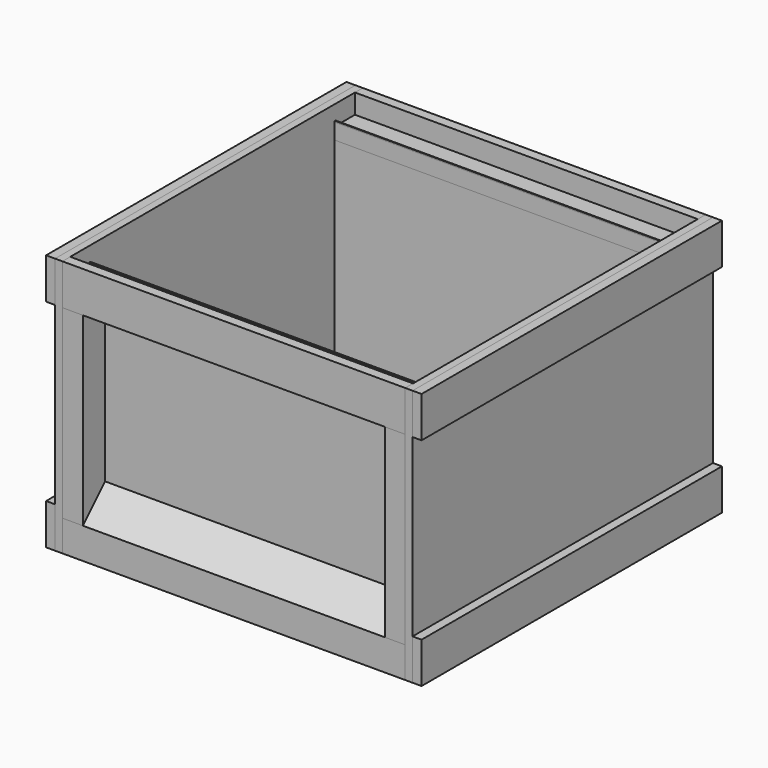
from build123d import *

# Parameters (mm, degrees)
F0_W      = 9
F0_H      = 291
F1_DEPTH  = 210
F2_W      = 34
F2_H      = 38
F3_DEPTH  = 210
F5_DEPTH  = 420
F9_DEPTH  = 9
F10_W     = 11
F10_H     = 50
F11_DEPTH = 460
F12_W     = 34
F12_H     = 227
F13_DEPTH = 25
F16_DEPTH = 370


# Not quite as in the source:
# - ends of sketch curves that miss each other by under 0.0002 mm in the source are joined


with BuildPart() as f1:
    # F0 (on Right) → F1 (new body, symmetric)
    with BuildSketch(Plane.YZ):
        with Locations((39.679, 143.4123)):
            Rectangle(F0_W, F0_H)
    extrude(amount=F1_DEPTH, both=True)


with BuildPart() as f1b:
    # F0 (on Right) → F1, piece 2 (new body, symmetric)
    with BuildSketch(Plane.YZ):
        Polygon((427.179, 288.9123), (418.179, 288.9123), (418.179, -2.0877000002), (427.1789405548, -2.0877634065), align=None)
    extrude(amount=F1_DEPTH, both=True)


with BuildPart() as f3:
    # F2 (on Right) → F3 (new body, symmetric)
    with BuildSketch(Plane.YZ):
        with Locations((18.179, 16.9123)):
            Rectangle(F2_W, F2_H)
    extrude(amount=F3_DEPTH, both=True)


with BuildPart() as f3b:
    # F2 (on Right) → F3, piece 2 (new body, symmetric)
    with BuildSketch(Plane.YZ):
        Polygon((13.179, 312.9123), (1.179, 312.9123), (1.179, 262.9123), (35.179, 262.9123), (35.179, 288.9123), (13.179, 288.9123), align=None)
    extrude(amount=F3_DEPTH, both=True)


with BuildPart() as f3c:
    # F2 (on Right) → F3, piece 3 (new body, symmetric)
    with BuildSketch(Plane.YZ):
        Polygon((461.179, 262.9123), (461.179, 312.9123), (449.179, 312.9123), (449.179, 288.9123), (427.179, 288.9123), (427.179, 262.9123), align=None)
    extrude(amount=F3_DEPTH, both=True)


with BuildPart() as f3d:
    # F2 (on Right) → F3, piece 4 (new body, symmetric)
    with BuildSketch(Plane.YZ):
        with Locations((444.179, 16.9123)):
            Rectangle(F2_W, F2_H)
    extrude(amount=F3_DEPTH, both=True)


with BuildPart() as f5:
    # F4 (on face) → F5 (new body, through all)
    with BuildSketch(Plane.YZ.offset(210)):
        with BuildLine():
            ThreePointArc((43.116056405, 294.2939847231), (43.7817730788, 294.4769973335), (44.179, 293.9123))
            Line((44.179, 293.9123), (44.179, 274.5123))
            Line((44.179, 274.5123), (44.729, 274.5123))
            Line((44.729, 274.5123), (44.729, 293.9123))
            ThreePointArc((44.729, 293.9123), (44.5195970607, 294.5739473149), (43.9676484011, 294.9946365559))
            Line((43.9676484011, 294.9946365559), (43.1903515989, 294.9946365559))
            ThreePointArc((43.1903515989, 294.9946365559), (42.9173526851, 294.8528970607), (42.6916914429, 294.6438623859))
            Line((42.6916914429, 294.6438623859), (38.2546350379, 289.2621776628))
            Line((38.2546350379, 289.2621776628), (38.679, 288.9123))
            Line((38.679, 288.9123), (43.116056405, 294.2939847231))
        make_face()
    extrude(amount=-F5_DEPTH)


with BuildPart() as f7_1:
    # F7: instance of F5
    add(f5.part.mirror(Plane(origin=(0, 231.179, 143.4122999999), x_dir=(-1, 0, 0), z_dir=(0, 1, 0))))


with BuildPart() as f9:
    # F8 (on face) → F9 (new body)
    with BuildSketch(Plane.YZ.offset(210)):
        Polygon((1.179, 312.9123), (1.179, -2.0877), (461.179, -2.0877), (461.179, 312.9123), (13.179, 312.9123), align=None)
    extrude(amount=F9_DEPTH)


with BuildPart() as f11:
    # F10 (on face) → F11 (new body, through all)
    with BuildSketch(Plane.XZ.offset(-1.179)):
        with Locations((224.5, 287.9123)):
            Rectangle(F10_W, F10_H)
    extrude(amount=-F11_DEPTH)


with BuildPart() as f11b:
    # F10 (on face) → F11, piece 2 (new body, through all)
    with BuildSketch(Plane.XZ.offset(-1.179)):
        with Locations((224.5, 22.9123)):
            Rectangle(F10_W, F10_H)
    extrude(amount=-F11_DEPTH)


with BuildPart() as f13:
    # F12 (on face) → F13 (new body)
    with BuildSketch(Plane(origin=(210, 0, 0), x_dir=(0, -1, 0), z_dir=(-1, 0, 0))):
        with Locations((-18.179, 149.4123)):
            Rectangle(F12_W, F12_H)
    extrude(amount=F13_DEPTH)


with BuildPart() as f13b:
    # F12 (on face) → F13, piece 2 (new body)
    with BuildSketch(Plane(origin=(210, 0, 0), x_dir=(0, -1, 0), z_dir=(-1, 0, 0))):
        with Locations((-444.179, 149.4123)):
            Rectangle(F12_W, F12_H)
    extrude(amount=F13_DEPTH)


with BuildPart() as f14_1:
    # F14: instance of F9
    add(f9.part.mirror(Plane.YZ))


with BuildPart() as f14_2:
    # F14: instance of F11b
    add(f11b.part.mirror(Plane.YZ))


with BuildPart() as f14_3:
    # F14: instance of F11
    add(f11.part.mirror(Plane.YZ))


with BuildPart() as f14_4:
    # F14: instance of F13
    add(f13.part.mirror(Plane.YZ))


with BuildPart() as f14_5:
    # F14: instance of F13b
    add(f13b.part.mirror(Plane.YZ))


with BuildPart() as f16:
    # F15 (on face) → F16 (new body, through all)
    with BuildSketch(Plane(origin=(185, 0, 0), x_dir=(0, -1, 0), z_dir=(-1, 0, 0))):
        Polygon((-35.179, 69.9123), (-35.179, 35.9123), (-1.179, 35.9123), align=None)
    extrude(amount=F16_DEPTH)


with BuildPart() as f16b:
    # F15 (on face) → F16, piece 2 (new body, through all)
    with BuildSketch(Plane(origin=(185, 0, 0), x_dir=(0, -1, 0), z_dir=(-1, 0, 0))):
        Polygon((-427.179, 35.9123), (-427.179, 69.9123), (-461.179, 35.9123), align=None)
    extrude(amount=F16_DEPTH)


solid = Compound([f1.part, f1b.part, f3.part, f3b.part, f3c.part, f3d.part, f5.part, f7_1.part, f9.part, f11.part, f11b.part, f13.part, f13b.part, f14_1.part, f14_2.part, f14_3.part, f14_4.part, f14_5.part, f16.part, f16b.part])
